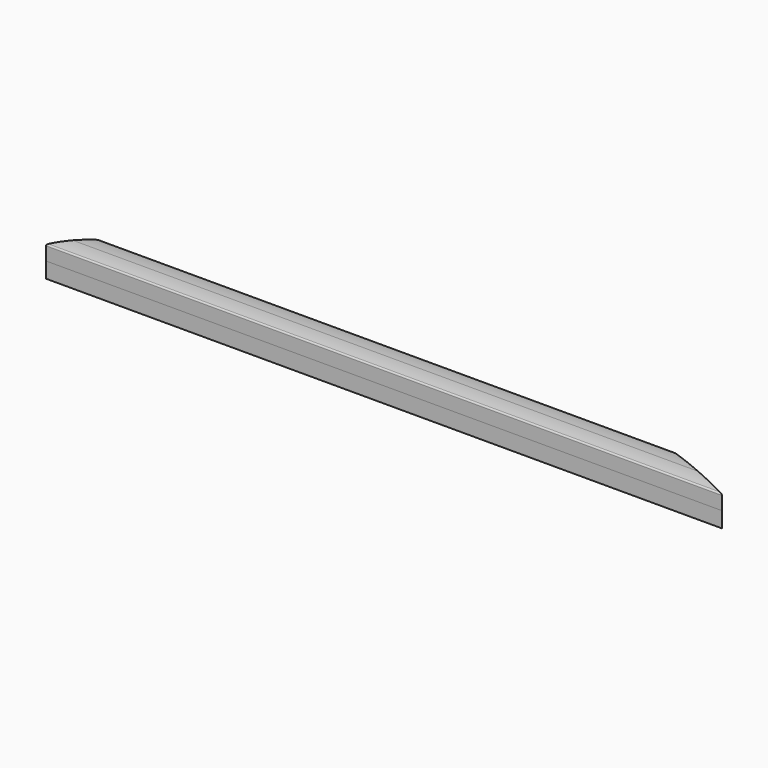
from build123d import *

# Parameters (mm, degrees)
F2_DEPTH      = 1000
F4_DEPTH      = 1000
F8_DEPTH      = 10.001
F8_DEPTH_BACK = 10.001


# Not quite as in the source:
# - ends of sketch curves that miss each other by under 0.0002 mm in the source are joined


with BuildPart() as f2:
    # F1 (on Right) → F2 (new body)
    with BuildSketch(Plane.YZ):
        with BuildLine():
            Line((0, -9), (0, -10))
            Line((0, -10), (10, -10))
            Line((10, -10), (10, -0.2))
            Line((10, -0.2), (9, -0.2))
            ThreePointArc((9, -0.2), (8.5, -0.7), (9, -1.2))
            ThreePointArc((9, -1.2), (9.5, -1.7), (9, -2.2))
            Line((9, -2.2), (9, -9))
            Line((9, -9), (0, -9))
        make_face()
    extrude(amount=F2_DEPTH)

    # F5: F2 across plane


with BuildPart() as f4:
    # F3 (on Right) → F4 (new body)
    with BuildSketch(Plane.YZ):
        with BuildLine():
            Line((9, -0.2), (10, -0.2))
            Line((10, -0.2), (10, 8.1663783152))
            ThreePointArc((10, 8.1663783152), (9.7693092582, 8.8052548802), (9.1836734694, 9.1493656277))
            ThreePointArc((9.1836734694, 9.1493656277), (4.6114920912, 9.7868872364), (0, 10))
            Line((0, 10), (0, 9))
            ThreePointArc((0, 9), (4.5192622493, 8.7911494917), (9, 8.1663783152))
            Line((9, 8.1663783152), (9, 0.8))
            ThreePointArc((9, 0.8), (7.5, -0.7), (9, -2.2))
            ThreePointArc((9, -2.2), (9.5, -1.7), (9, -1.2))
            ThreePointArc((9, -1.2), (8.5, -0.7), (9, -0.2))
        make_face()
    extrude(amount=F4_DEPTH)

    # F6: F4 across plane


with BuildPart() as f2_1:
    add(f2.part)
    add(f2.part.mirror(Plane.XZ))


with BuildPart() as f4_1:
    add(f4.part)
    add(f4.part.mirror(Plane.XZ))


with BuildPart() as f8_tool:
    # F7 (on Top) → F8 (new body, two sides)
    with BuildSketch(Plane.XY) as f8_sk:
        Polygon((0, 10), (0, 0), (0, -10), (17.3857347563, 10), align=None)
        Polygon((378.0031490553, 10), (424, -10), (1016.9613361359, -10), (1016.9613361359, 10), (709.9114895723, 10), align=None)
    extrude(amount=F8_DEPTH)
    extrude(f8_sk.sketch, amount=-F8_DEPTH_BACK)


with BuildPart() as f2_2:
    add(f2_1.part)

    # F8: cut by f8_tool
    add(f8_tool.part, mode=Mode.SUBTRACT)


with BuildPart() as f4_2:
    add(f4_1.part)

    # F8: cut by f8_tool
    add(f8_tool.part, mode=Mode.SUBTRACT)


solid = Compound([f2_2.part, f4_2.part])
